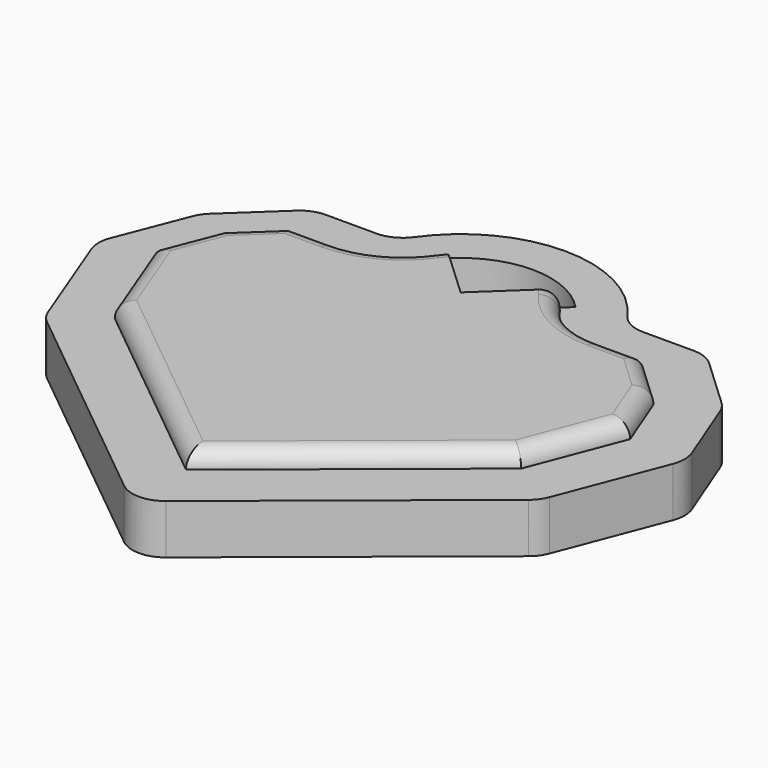
from build123d import *

# Parameters (mm, degrees)
F1_DEPTH = 1.5
F2_R     = 1
F3_R     = 1
F5_DEPTH = 0.5
F6_R     = 0.49999


# Not quite as in the source:
# - a fillet or chamfer is up to 0.001 mm smaller than in the source, because OpenCascade refuses the exact size


with BuildPart() as f1:
    # F0 (on Top) → F1 (new body)
    with BuildSketch(Plane.XY):
        with BuildLine():
            ThreePointArc((-1.986540854, 9.3519296497), (0, 10.2135319331), (1.986540854, 9.3519296497))
            Line((1.986540854, 9.3519296497), (3.4759494504, 9.3519296497))
            ThreePointArc((3.4759494504, 9.3519296497), (0, 11.4346017651), (-3.4759494504, 9.3519296497))
            Line((-3.4759494504, 9.3519296497), (-1.986540854, 9.3519296497))
        make_face()
        with BuildLine():
            Line((5.9530865401, 9.3519296497), (3.4759494504, 9.3519296497))
            ThreePointArc((3.4759494504, 9.3519296497), (3.8237056455, 8.4510290854), (3.9419905804, 7.4926111847))
            ThreePointArc((3.9419905804, 7.4926111847), (-0.9584179006, 3.6689055392), (-3.4759494504, 9.3519296497))
            Line((-3.4759494504, 9.3519296497), (-5.9530865401, 9.3519296497))
            Line((-5.9530865401, 9.3519296497), (-7.8950412571, 7.5339297764))
            Line((-7.8950412571, 7.5339297764), (-8.927995339, 4.88956552))
            Line((-8.927995339, 4.88956552), (-7.4818595313, 1.1296109296))
            Line((-7.4818595313, 1.1296109296), (0, -4.9441619776))
            Line((0, -4.9441619776), (7.4818595313, 1.1296109296))
            Line((7.4818595313, 1.1296109296), (8.927995339, 4.88956552))
            Line((8.927995339, 4.88956552), (7.8950412571, 7.5339297764))
            Line((7.8950412571, 7.5339297764), (5.9530865401, 9.3519296497))
        make_face()
        with BuildLine():
            Line((3.4759494504, 9.3519296497), (1.986540854, 9.3519296497))
            ThreePointArc((1.986540854, 9.3519296497), (2.5306748058, 8.4921584552), (2.7209207483, 7.4926111847))
            ThreePointArc((2.7209207483, 7.4926111847), (-0.9995472705, 4.9619363789), (-1.986540854, 9.3519296497))
            Line((-1.986540854, 9.3519296497), (-3.4759494504, 9.3519296497))
            ThreePointArc((-3.4759494504, 9.3519296497), (-0.9584179006, 3.6689055392), (3.9419905804, 7.4926111847))
            ThreePointArc((3.9419905804, 7.4926111847), (3.8237056455, 8.4510290854), (3.4759494504, 9.3519296497))
        make_face()
        with BuildLine():
            Line((1.986540854, 9.3519296497), (0, 7.4926111847))
            Line((0, 7.4926111847), (-1.986540854, 9.3519296497))
            ThreePointArc((-1.986540854, 9.3519296497), (-0.9995472705, 4.9619363789), (2.7209207483, 7.4926111847))
            ThreePointArc((2.7209207483, 7.4926111847), (2.5306748058, 8.4921584552), (1.986540854, 9.3519296497))
        make_face()
    extrude(amount=F1_DEPTH)

    # F2
    f2_edges = [f1.edges().sort_by_distance(p)[0] for p in [
        (0, -4.944162, 0.75),
    ]]
    fillet(f2_edges, radius=F2_R)

    # F3
    f3_edges = [f1.edges().sort_by_distance(p)[0] for p in [
        (7.48186, 1.129611, 0.75),
        (8.927995, 4.889566, 0.75),
        (7.895041, 7.53393, 0.75),
        (5.953087, 9.35193, 0.75),
        (-7.48186, 1.129611, 0.75),
        (-8.927995, 4.889566, 0.75),
        (-7.895041, 7.53393, 0.75),
        (-5.953087, 9.35193, 0.75),
        (-3.475949, 9.35193, 0.75),
        (3.475949, 9.35193, 0.75),
    ]]
    fillet(f3_edges, radius=F3_R)

    # F4 (on face) → F5 (join)
    with BuildSketch(Plane.XY.offset(1.5)):
        with BuildLine():
            ThreePointArc((-1.7098843542, 9.0929908328), (-1.8141917234, 8.9737012946), (-1.9101937031, 8.8476313097))
            ThreePointArc((-1.9101937031, 8.8476313097), (-2.837339859, 8.0420404539), (-4.0308273111, 7.7519295737))
            Line((-4.0308273111, 7.7519295737), (-5.3210256953, 7.7519295737))
            Line((-5.3210256953, 7.7519295737), (-6.5367130105, 6.613839501))
            Line((-6.5367130105, 6.613839501), (-7.2120080925, 4.88508291))
            Line((-7.2120080925, 4.88508291), (-6.141831705, 2.1026231998))
            Line((-6.141831705, 2.1026231998), (0, -2.8833152363))
            Line((0, -2.8833152363), (6.141831705, 2.1026231998))
            Line((6.141831705, 2.1026231998), (7.2120080925, 4.88508291))
            Line((7.2120080925, 4.88508291), (6.5367130105, 6.613839501))
            Line((6.5367130105, 6.613839501), (5.3210256953, 7.7519295737))
            Line((5.3210256953, 7.7519295737), (4.0308273111, 7.7519295737))
            ThreePointArc((4.0308273111, 7.7519295737), (2.837339859, 8.0420404539), (1.9101937031, 8.8476313097))
            ThreePointArc((1.9101937031, 8.8476313097), (1.8141917234, 8.9737012946), (1.7098843542, 9.0929908328))
            Line((1.7098843542, 9.0929908328), (0, 7.4926111847))
            Line((0, 7.4926111847), (-1.7098843542, 9.0929908328))
        make_face()
    extrude(amount=F5_DEPTH)

    # F6 (radius 0.5 in the source; OpenCascade refuses exactly that, so slightly less here)
    f6_edges = [f1.edges().sort_by_distance(p)[0] for p in [
        (-5.928869, 7.182885, 2),
        (-6.874361, 5.749461, 2),
        (-6.67692, 3.493853, 2),
        (-3.070916, -0.390346, 2),
        (3.070916, -0.390346, 2),
        (6.67692, 3.493853, 2),
        (6.874361, 5.749461, 2),
        (5.928869, 7.182885, 2),
        (4.675927, 7.75193, 2),
        (2.83734, 8.04204, 2),
        (-2.83734, 8.04204, 2),
    ]]
    fillet(f6_edges, radius=F6_R)


solid = f1.part
